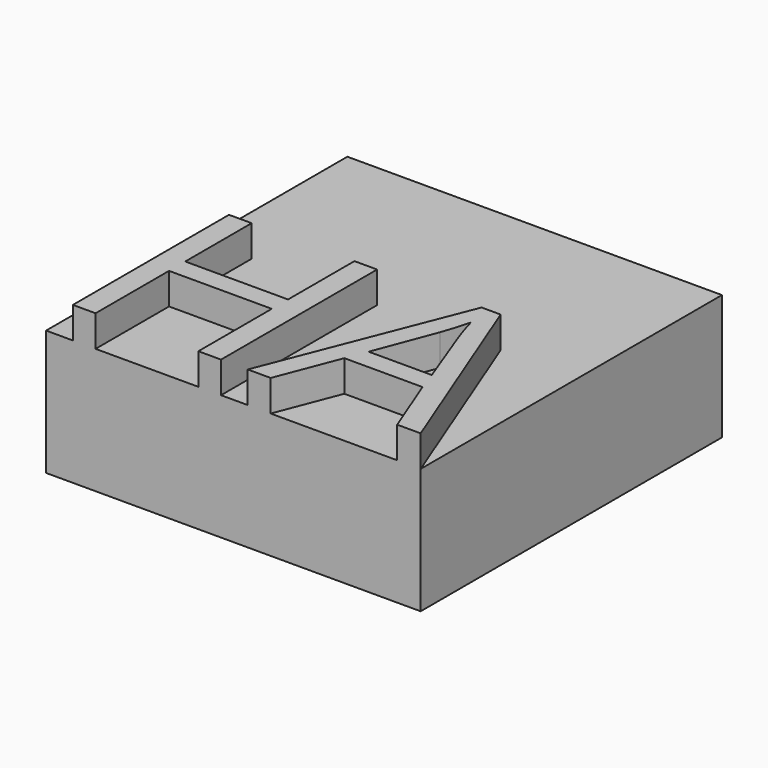
from build123d import *

# Parameters (mm, degrees)
F0_W         = 75.9043246508
F0_H         = 76.3113349676
F1_DEPTH     = 25.4
F2_TEXT_SIZE = 55.3793522304
F3_DEPTH     = 6.35


# Not quite as in the source:
# - Text() gives the source's letters only with a copy of the font that has no kerning and outlines rounded to 1/6400 em; it was checked with that copy


with BuildPart() as f1:
    # F0 (on Top) → F1 (new body)
    with BuildSketch(Plane.XY):
        with Locations((-37.9521623254, 38.1556674838)):
            Rectangle(F0_W, F0_H)
    extrude(amount=F1_DEPTH)

    # F2 (on face) → F3 (join)
    with BuildSketch(Plane.XY.offset(25.4)):
        with Locations((-75.9043246508, 0)):
            Text('HA', F2_TEXT_SIZE, font='Open Sans', text_align=(TextAlign.LEFT, TextAlign.BOTTOM))
    extrude(amount=F3_DEPTH)


solid = f1.part
